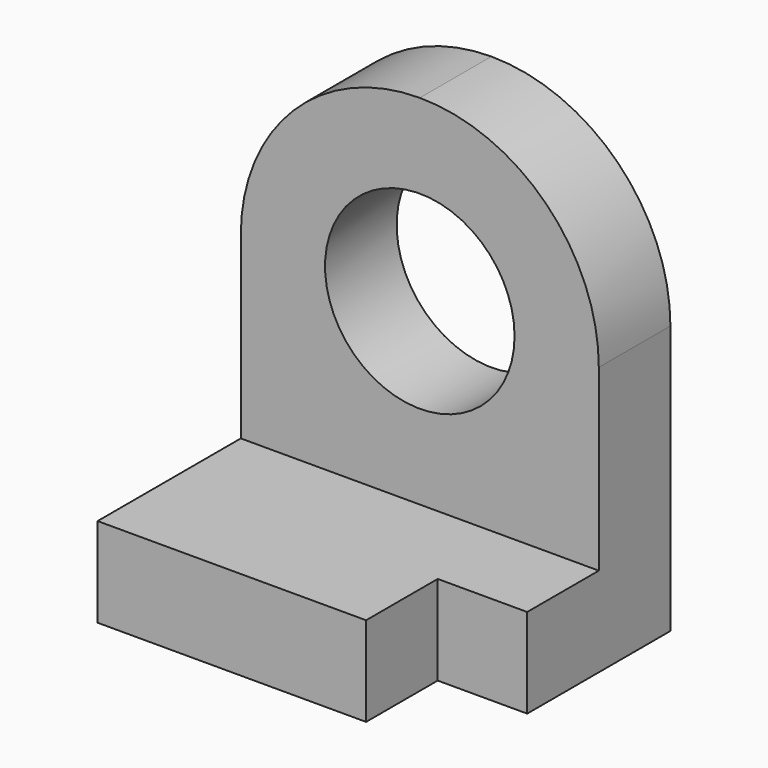
from build123d import *

# Parameters (mm, degrees)
F0_W     = 101.6
F0_H     = 76.2
F1_DEPTH = 25.4
F2_W     = 25.4
F2_H     = 25.4
F3_DEPTH = 25.401
F4_W     = 101.6
F4_H     = 25.4
F5_DEPTH = 101.6
F6_R     = 50.8
F7_R     = 50.79999
F8_R     = 26.8874983084
F9_DEPTH = 25.401


# Not quite as in the source:
# - a fillet or chamfer is up to 0.001 mm smaller than in the source, because OpenCascade refuses the exact size


with BuildPart() as f1:
    # F0 (on Top) → F1 (new body)
    with BuildSketch(Plane.XY):
        Rectangle(F0_W, F0_H)
    extrude(amount=F1_DEPTH)

    # F2 (on face) → F3 (cut, through all)
    with BuildSketch(Plane.XY.offset(25.4)):
        with Locations((38.1, -25.4)):
            Rectangle(F2_W, F2_H)
    extrude(amount=-F3_DEPTH, mode=Mode.SUBTRACT)

    # F4 (on face) → F5 (join)
    with BuildSketch(Plane.XY.offset(25.4)):
        with Locations((0, 25.4)):
            Rectangle(F4_W, F4_H)
    extrude(amount=F5_DEPTH)

    # F6
    f6_edges = [f1.edges().sort_by_distance(p)[0] for p in [
        (-50.8, 25.4, 127),
    ]]
    fillet(f6_edges, radius=F6_R)

    # F7 (radius 50.8 in the source; OpenCascade refuses exactly that, so slightly less here)
    f7_edges = [f1.edges().sort_by_distance(p)[0] for p in [
        (50.8, 25.4, 127),
    ]]
    fillet(f7_edges, radius=F7_R)

    # F8 (on face) → F9 (cut, through all)
    with BuildSketch(Plane.XZ.offset(-12.7)):
        with Locations((0, 76.2)):
            Circle(F8_R)
    extrude(amount=-F9_DEPTH, mode=Mode.SUBTRACT)


solid = f1.part
